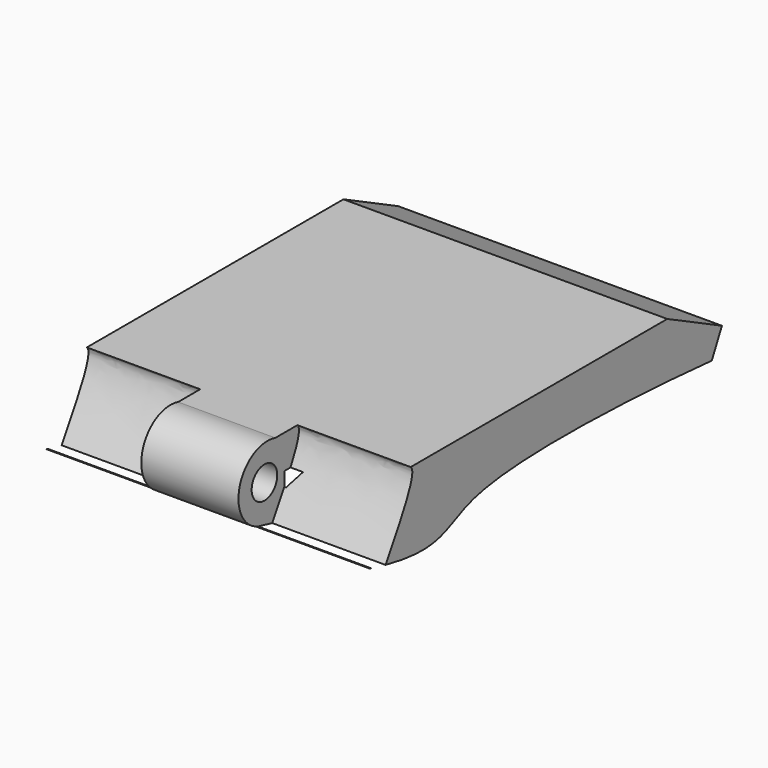
from build123d import *

# Parameters (mm, degrees)
F1_DEPTH = 50
F0_R     = 4.94
F2_R     = 4.94
F3_DEPTH = 35
F5_DEPTH = 25


# Not quite as in the source:
# - a pattern or mirror of a feature is missing from the dataset's text; its kind, count and spacing are read off the source's solid


with BuildPart() as f1:
    # F0 (on Right) → F1 (new body, symmetric)
    with BuildSketch(Plane.YZ):
        with BuildLine():
            add(Edge.make_bspline(
                [(-3.0323168048, -10.8181582689), (-2.8424272556, -10.8663900835), (-2.6538250298, -10.9140078026), (-2.4664978488, -10.9610164628)],
                knots=[0, 0, 0, 0, 0.0026237907, 0.0026237907, 0.0026237907, 0.0026237907], degree=3))
            ThreePointArc((-3.0323168048, -10.8181582689), (-2.7503350277, -10.8932617141), (-2.4664978488, -10.9610164628))
        make_face()
    extrude(amount=F1_DEPTH, both=True)


with BuildPart() as f1b:
    # F0 (on Right) → F1, piece 2 (new body, symmetric)
    with BuildSketch(Plane.YZ):
        with BuildLine():
            ThreePointArc((4.1932159041, 10.4232640722), (-9.5274989599, 2.9671522383), (-2.4664978488, -10.9610164628))
            add(Edge.make_bspline(
                [(-2.4664978488, -10.9610164628), (25.9397967098, -18.0894099096), (23.6511889197, -0.8509774431), (106.1659529805, -5.9674950317), (128.9111768297, -7.8934305644)],
                knots=[0.0026237907, 0.0026237907, 0.0026237907, 0.0026237907, 0.4004954175, 1, 1, 1, 1], degree=3))
            Line((128.9111768297, -7.8934305644), (132.8115165234, 0))
            Line((132.8115165234, 0), (111.7171202219, 10.4232640722))
            Line((111.7171202219, 10.4232640722), (4.1932159041, 10.4232640722))
        make_face()
        Circle(F0_R, mode=Mode.SUBTRACT)
    extrude(amount=F1_DEPTH, both=True)

    # F2 (on face) → F3 (cut)
    with BuildSketch(Plane.YZ.offset(50)):
        with BuildLine():
            Line((6.8677525204, 10.4232640722), (4.1932159041, 10.4232640722))
            ThreePointArc((4.1932159041, 10.4232640722), (-0.1693274921, 10.7589359529), (-4.3277336512, 9.3980102714))
            add(Edge.make_bspline(
                [(6.8677525204, 10.4232640722), (3.5056440269, 9.7988076387), (-0.669971735, 8.8655469209), (-4.3277336512, 9.3980102714)],
                knots=[0.4757656296, 0.4757656296, 0.4757656296, 0.4757656296, 0.6363648624, 0.6363648624, 0.6363648624, 0.6363648624], degree=3))
        make_face()
        with BuildLine():
            add(Edge.make_bspline(
                [(12.6898856834, 10.4232640722), (11.721497416, 11.2240656804), (9.5543495494, 10.9222553456), (6.8677525204, 10.4232640722)],
                knots=[0.3474338334, 0.3474338334, 0.3474338334, 0.3474338334, 0.4757656296, 0.4757656296, 0.4757656296, 0.4757656296], degree=3))
            Line((6.8677525204, 10.4232640722), (12.6898856834, 10.4232640722))
        make_face()
        with BuildLine():
            Line((12.6898856834, 10.4232640722), (6.8677525204, 10.4232640722))
            add(Edge.make_bspline(
                [(6.8677525204, 10.4232640722), (3.5056440269, 9.7988076387), (-0.669971735, 8.8655469209), (-4.3277336512, 9.3980102714)],
                knots=[0.4757656296, 0.4757656296, 0.4757656296, 0.4757656296, 0.6363648624, 0.6363648624, 0.6363648624, 0.6363648624], degree=3))
            ThreePointArc((-4.3277336512, 9.3980102714), (-9.9876923855, -1.3840180073), (-2.4664978488, -10.9610164628))
            add(Edge.make_bspline(
                [(-2.4664978488, -10.9610164628), (-0.516074965, -11.4504636758), (1.2961245634, -11.8738848534), (2.9839597919, -12.2369650055)],
                knots=[0.0026237907, 0.0026237907, 0.0026237907, 0.0026237907, 0.0299423107, 0.0299423107, 0.0299423107, 0.0299423107], degree=3))
            add(Edge.make_bspline(
                [(2.9839597919, -12.2369650055), (9.1470031068, -1.994389644), (15.3116120056, 8.255246629), (12.6898856834, 10.4232640722)],
                knots=[0, 0, 0, 0, 0.3474338334, 0.3474338334, 0.3474338334, 0.3474338334], degree=3))
        make_face()
        Circle(F2_R, mode=Mode.SUBTRACT)
        Circle(F2_R)
    f3 = extrude(amount=-F3_DEPTH, mode=Mode.SUBTRACT)

    # F3_copies: F3 across plane
    add(f3.mirror(Plane(origin=(-1.2e-05, 0, 0), x_dir=(0, 0, -1), z_dir=(-1, 0, 0))), mode=Mode.SUBTRACT)

    # F4 (on Top) → F5 (cut)
    with BuildSketch(Plane.XY):
        with BuildLine():
            Line((-46.2965779006, 29.526354745), (-15.5149381608, 7.6813208871))
            Line((-15.5149381608, 7.6813208871), (15.5149381608, 7.6813208871))
            Line((15.5149381608, 7.6813208871), (46.2965779006, 29.526354745))
            Line((46.2965779006, 29.526354745), (47.0022331808, 120.5560959189))
            ThreePointArc((47.0022331808, 120.5560959189), (45.5515940339, 124.1166584252), (42.0023834047, 125.5948543549))
            Line((42.0023834047, 125.5948543549), (-41.2965779006, 125.5948543549))
            ThreePointArc((-41.2965779006, 125.5948543549), (-44.8321118066, 124.1303882608), (-46.2965779006, 120.5948543549))
            Line((-46.2965779006, 120.5948543549), (-46.2965779006, 29.526354745))
        make_face()
    extrude(amount=-F5_DEPTH, mode=Mode.SUBTRACT)


solid = Compound([f1.part, f1b.part])
